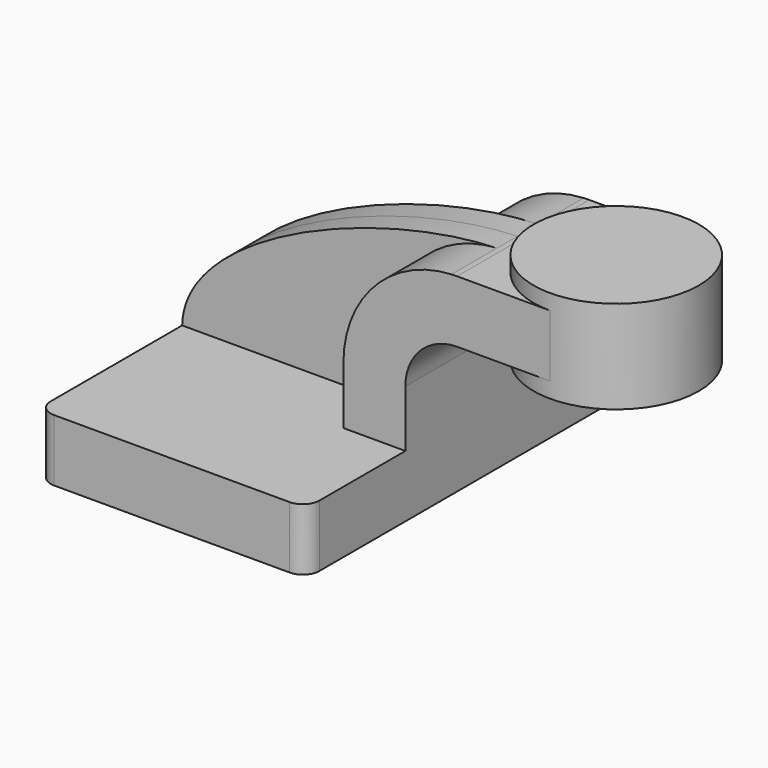
from build123d import *

# Parameters (mm, degrees)
F1_DEPTH = 63.5
F0_W     = 25.4
F0_H     = 19.05
F2_DEPTH = 25.4
F3_DEPTH = 7.9375
F5_R     = 5.08


# Not quite as in the source:
# - ends of sketch curves that miss each other by under 0.0002 mm in the source are joined


with BuildPart() as f1:
    # F0 (on Front) → F1 (new body, symmetric)
    with BuildSketch(Plane.XZ):
        Polygon((-41.275, -9.525), (41.275, -9.525), (41.275, 9.525), (22.225, 9.525), (-41.275, 9.525), align=None)
    extrude(amount=F1_DEPTH, both=True)

    # F0 (on Front) → F2 (join, symmetric)
    with BuildSketch(Plane.XZ):
        with BuildLine():
            Line((22.225, 9.525), (41.275, 9.525))
            Line((41.275, 9.525), (41.275, 27.0002))
            ThreePointArc((41.275, 27.0002), (45.9246798487, 38.2255201513), (57.15, 42.8752))
            Line((57.15, 42.8752), (60.325, 42.8752))
            Line((60.325, 42.8752), (60.325, 61.9252))
            Line((60.325, 61.9252), (57.15, 61.9252))
            add(Edge.make_bspline(
                [(55.4308013552, 61.8828601769), (56.0086976587, 61.9022725241), (56.5818561966, 61.916408872), (57.15, 61.9252)],
                knots=[109.8295826069, 109.8295826069, 109.8295826069, 109.8295826069, 111.5045361635, 111.5045361635, 111.5045361635, 111.5045361635], degree=3))
            ThreePointArc((55.4308013552, 61.8828601769), (31.8537686832, 51.0804056919), (22.225, 27.0002))
            Line((22.225, 27.0002), (22.225, 9.525))
        make_face()
        with Locations((73.025, 52.4002)):
            Rectangle(F0_W, F0_H)
    extrude(amount=F2_DEPTH, both=True)

    # F0 (on Front) → F3 (join, symmetric)
    with BuildSketch(Plane.XZ):
        with BuildLine():
            add(Edge.make_bspline(
                [(-41.275, 9.525), (-40.7272405937, 36.6521064094), (17.5371477958, 60.609959217), (55.4308013552, 61.8828601769)],
                knots=[0, 0, 0, 0, 109.8295826069, 109.8295826069, 109.8295826069, 109.8295826069], degree=3))
            Line((-41.275, 9.525), (22.225, 9.525))
            Line((22.225, 9.525), (22.225, 27.0002))
            ThreePointArc((22.225, 27.0002), (31.8537686832, 51.0804056919), (55.4308013552, 61.8828601769))
        make_face()
    extrude(amount=F3_DEPTH, both=True)

    # F0 (on Front) → F4 (revolve)
    with BuildSketch(Plane.XZ):
        Polygon((85.725, 61.9252), (85.725, 42.8752), (85.725, 38.1), (111.125, 38.1), (111.125, 66.675), (85.725, 66.675), align=None)
    revolve(axis=Axis((85.725, 0, 52.3875), (0, 0, -1)))

    # F5
    f5_edges = [f1.edges().sort_by_distance(p)[0] for p in [
        (41.275, -63.5, 0),
        (-41.275, -63.5, 0),
        (-41.275, 63.5, 0),
        (41.275, 63.5, 0),
    ]]
    fillet(f5_edges, radius=F5_R)


solid = f1.part
